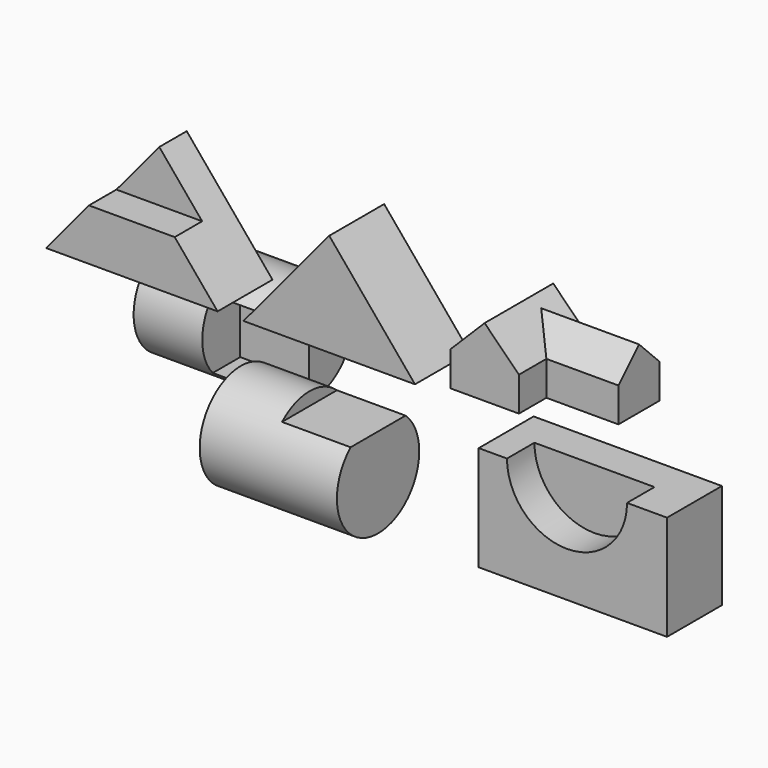
from build123d import *

# Parameters (mm, degrees)
F1_DEPTH  = 101.6
F3_DEPTH  = 50.8
F5_DEPTH  = 101.6
F7_DEPTH  = 127
F8_DEPTH  = 127
F12_R     = 76.2
F13_DEPTH = 203.2
F15_DEPTH = 101.6
F17_R     = 76.2
F18_DEPTH = 203.2
F20_DEPTH = 101.6
F21_W     = 278.8744270802
F21_H     = 155.3969010711
F22_DEPTH = 101.6
F24_DEPTH = 50.8


with BuildPart() as f1:
    # F0 (on Front) → F1 (new body)
    with BuildSketch(Plane.XZ):
        Polygon((-165.3565709478, 152.4), (-292.3565709478, 0), (-38.3565709478, 0), align=None)
    extrude(amount=F1_DEPTH)

    # F2 (on face) → F3 (cut)
    with BuildSketch(Plane.XZ.offset(101.6)):
        Polygon((-165.3565709478, 152.4), (-228.8565709478, 76.2), (-101.8565709478, 76.2), align=None)
    extrude(amount=-F3_DEPTH, mode=Mode.SUBTRACT)


with BuildPart() as f5:
    # F4 (on Front) → F5 (new body)
    with BuildSketch(Plane.XZ):
        Polygon((127, 152.4), (0, 0), (254, 0), align=None)
    extrude(amount=F5_DEPTH)


with BuildPart() as f7:
    # F6 (on Front) → F7 (new body)
    with BuildSketch(Plane.XZ):
        Polygon((326.6123191833, 79.5415978638), (326.6123191833, 28.7415978638), (428.2123191833, 28.7415978638), (428.2123191833, 79.5415978638), (377.4123191833, 130.3415978638), align=None)
    extrude(amount=F7_DEPTH)

    # F6 (on Front) → F8 (join)
    with BuildSketch(Plane.XZ):
        Polygon((326.6123191833, 79.5415978638), (326.6123191833, 28.7415978638), (428.2123191833, 28.7415978638), (428.2123191833, 79.5415978638), (377.4123191833, 130.3415978638), align=None)
    extrude(amount=F8_DEPTH)

    # F10 (on offset) → F11 (join, up to the next surface of F7)
    with BuildSketch(Plane.YZ.offset(534.8923191833)):
        Polygon((-76.2, 28.7415978638), (0, 28.7415978638), (0, 79.5415978638), (-38.1, 117.6415978638), (-76.2, 79.5415978638), align=None)
    extrude(until=Until.NEXT, dir=(-1, 0, 0))


with BuildPart() as f13:
    # F12 (on Right) → F13 (new body)
    with BuildSketch(Plane.YZ):
        with Locations((-106.4828932285, -132.7566355467)):
            Circle(F12_R)
    extrude(amount=F13_DEPTH)

    # F14 (on face) → F15 (cut)
    with BuildSketch(Plane.YZ.offset(203.2)):
        with BuildLine():
            ThreePointArc((-55.6828932285, -75.9605089182), (-106.4828932285, -56.5566355467), (-157.2828932285, -75.9605089182))
            Line((-157.2828932285, -75.9605089182), (-55.6828932285, -75.9605089182))
        make_face()
    extrude(amount=-F15_DEPTH, mode=Mode.SUBTRACT)


with BuildPart() as f18:
    # F17 (on offset) → F18 (new body)
    with BuildSketch(Plane.YZ.offset(-288.544)):
        with Locations((131.9538205862, -149.6339142323)):
            Circle(F17_R)
    extrude(amount=F18_DEPTH)

    # F19 (on face) → F20 (cut)
    with BuildSketch(Plane.YZ.offset(-85.344)):
        with BuildLine():
            Line((125.9576939577, -98.8339142323), (75.1576939577, -98.8339142323))
            ThreePointArc((75.1576939577, -98.8339142323), (55.7538205862, -149.6339142323), (75.1576939577, -200.4339142323))
            Line((75.1576939577, -200.4339142323), (125.9576939577, -200.4339142323))
            Line((125.9576939577, -200.4339142323), (125.9576939577, -98.8339142323))
        make_face()
    extrude(amount=-F20_DEPTH, mode=Mode.SUBTRACT)


with BuildPart() as f22:
    # F21 (on Front) → F22 (new body)
    with BuildSketch(Plane.XZ):
        with Locations((487.779006362, -130.1811523736)):
            Rectangle(F21_W, F21_H)
    extrude(amount=F22_DEPTH)

    # F23 (on face) → F24 (cut)
    with BuildSketch(Plane.XZ.offset(101.6)):
        with BuildLine():
            ThreePointArc((390.1701270103, -52.482701838), (479.0701270103, -141.382701838), (567.9701270103, -52.482701838))
            Line((567.9701270103, -52.482701838), (390.1701270103, -52.482701838))
        make_face()
        with BuildLine():
            Line((390.1701270103, -52.482701838), (567.9701270103, -52.482701838))
            ThreePointArc((567.9701270103, -52.482701838), (479.0701270103, 36.417298162), (390.1701270103, -52.482701838))
        make_face()
    extrude(amount=-F24_DEPTH, mode=Mode.SUBTRACT)


solid = Compound([f1.part, f5.part, f7.part, f13.part, f18.part, f22.part])
